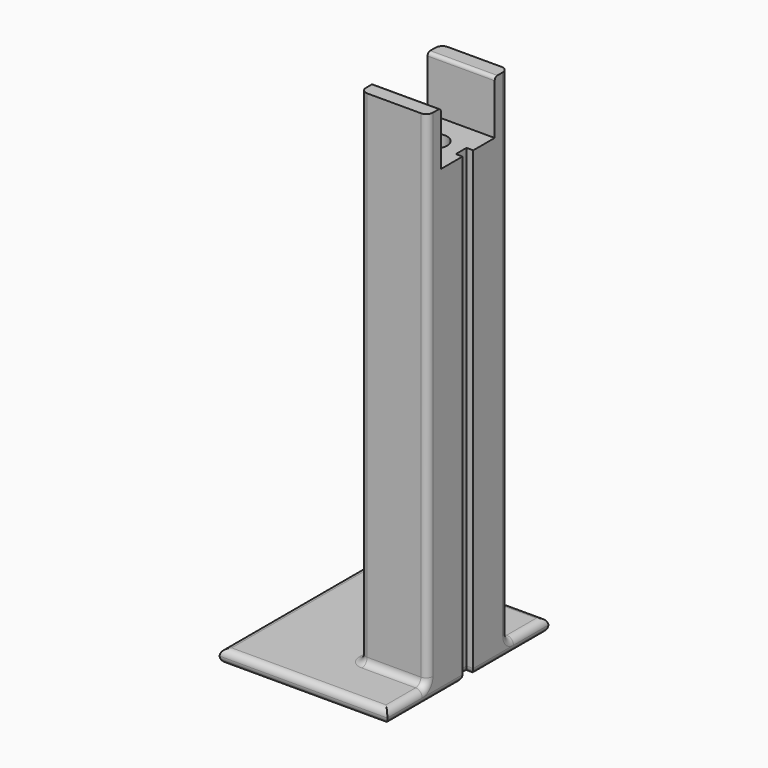
from build123d import *

# Parameters (mm, degrees)
F1_DEPTH     = 2
F2_R         = 1.9
F3_DEPTH     = 75
F4_W         = 10
F4_H         = 10
F5_DEPTH     = 8
F6_TEXT_SIZE = 13.8888888889
F7_DEPTH     = 0.5
F8_R         = 0.99999
F9_R         = 0.5


# Not quite as in the source:
# - a fillet or chamfer is up to 0.001 mm smaller than in the source, because OpenCascade refuses the exact size
# - Text() gives the source's letters only with a copy of the font that has no kerning and outlines rounded to 1/6400 em; it was checked with that copy


with BuildPart() as f1:
    # F0 (on Top) → F1 (new body)
    with BuildSketch(Plane.XY):
        Polygon((0, 1), (0, 15), (-25, 15), (-25, -15), (0, -15), (0, -1), (-1, -1), (-1, 1), align=None)
    extrude(amount=F1_DEPTH)

    # F2 (on face) → F3 (join)
    with BuildSketch(Plane.XY.offset(2)):
        Polygon((-1, 1), (0, 1), (0, 7.5), (-10, 7.5), (-10, -7.5), (0, -7.5), (0, -1), (-1, -1), align=None)
        with Locations((-5, 0)):
            Circle(F2_R, mode=Mode.SUBTRACT)
    extrude(amount=F3_DEPTH)

    # F4 (on face) → F5 (cut)
    with BuildSketch(Plane.XY.offset(77)):
        with Locations((-5, 0)):
            Rectangle(F4_W, F4_H)
    extrude(amount=-F5_DEPTH, mode=Mode.SUBTRACT)

    # F6 (on face) → F7 (cut)
    with BuildSketch(Plane(origin=(-10, 0, 0), x_dir=(0, -1, 0), z_dir=(-1, 0, 0))):
        with Locations(Location((-5, 68), (0, 0, -90))):
            Text('US holder', F6_TEXT_SIZE, font='Open Sans', text_align=(TextAlign.LEFT, TextAlign.BOTTOM))
    extrude(amount=-F7_DEPTH, mode=Mode.SUBTRACT)

    # F8 (radius 1 in the source; OpenCascade refuses exactly that, so slightly less here)
    f8_edges = [f1.edges().sort_by_distance(p)[0] for p in [
        (-10, -7.5, 39.5),
        (0, -7.5, 39.5),
        (-10, 7.5, 39.5),
        (0, 7.5, 39.5),
        (-5, 7.5, 2),
        (-10, 0, 2),
        (-5, -7.5, 2),
        (0, -11.25, 2),
        (-12.5, -15, 2),
        (-25, 0, 2),
        (-12.5, 15, 2),
        (0, 11.25, 2),
        (0, 8, 0),
        (-12.5, 15, 0),
        (-25, 0, 0),
        (-12.5, -15, 0),
        (0, -8, 0),
        (-0.5, -1, 0),
        (-1, 0, 0),
        (-0.5, 1, 0),
    ]]
    fillet(f8_edges, radius=F8_R)

    # F9
    f9_edges = [f1.edges().sort_by_distance(p)[0] for p in [
        (-5, 5, 77),
        (-5, -5, 77),
    ]]
    fillet(f9_edges, radius=F9_R)


solid = f1.part
